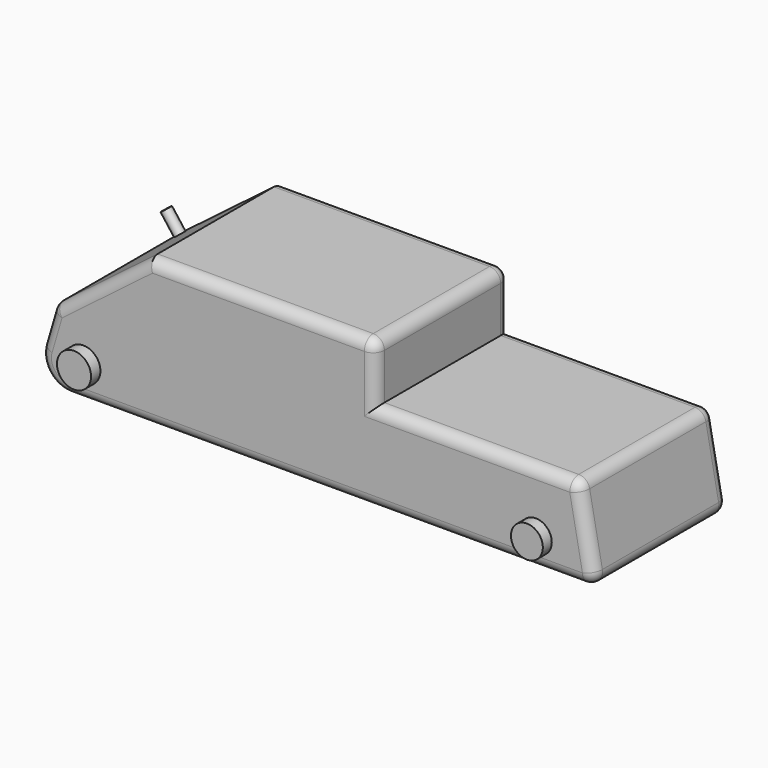
from build123d import *

# Parameters (mm, degrees)
F1_DEPTH    = 76.2
F2_R        = 5.08
F3_T1_DEPTH = 76.2
F3_T4_ANGLE = 106.3398594687
F3_T6_ANGLE = 106.3398594687
F4_R        = 7.7543468395
F5_DEPTH    = 0.254
F6_DEPTH    = 5.08
F7_R        = 7.6382634684
F8_DEPTH    = 5.08
F10_R       = 7.2706121331
F11_DEPTH   = 5.08
F9_R        = 7.2450103535
F12_DEPTH   = 5.08
F13_R       = 2.3168995741
F14_DEPTH   = 10.16


# Not quite as in the source:
# - a fillet or chamfer that OpenCascade refuses, or shapes differently, is made with other operations: its cross-section is extruded or revolved along the edge and cut away or added
# - the program builds the solid bodies; features that only make, move or delete a surface that nothing else refers to are left out


with BuildPart() as f1:
    # F0 (on Front) → F1 (new body)
    with BuildSketch(Plane.XZ):
        Polygon((-120.808057487, 0), (-130.5492073298, -33.2263112068), (126.3735592365, -33.2263112068), (118.6618208885, 7.3618022725), (26.1209160089, 7.3618022725), (26.1209160089, 33.3381965756), (-76.9728943706, 33.3381965756), align=None)
    extrude(amount=F1_DEPTH)

    # F2
    f2_edges = [f1.edges().sort_by_distance(p)[0] for p in [
        (-125.678632, -76.2, -16.613156),
        (-98.890476, -76.2, 16.669098),
        (-25.425989, -76.2, 33.338197),
        (26.120916, -76.2, 20.349999),
        (26.120916, 0, 20.349999),
        (26.120916, -38.1, 33.338197),
        (-98.890476, 0, 16.669098),
        (-25.425989, 0, 33.338197),
        (-125.678632, 0, -16.613156),
        (-2.087824, 0, -33.226311),
        (-120.808057, -38.1, 0),
        (-2.087824, -76.2, -33.226311),
        (72.391368, -76.2, 7.361802),
        (118.661821, -38.1, 7.361802),
        (122.51769, -76.2, -12.932254),
        (126.373559, -38.1, -33.226311),
        (122.51769, 0, -12.932254),
        (72.391368, 0, 7.361802),
    ]]
    fillet(f2_edges, radius=F2_R)

    # F3: fillet of radius 12.7 on 1 edges, made by hand

    # F3_s2 → F3_t1 (cut)
    with BuildSketch(Plane.XZ):
        with BuildLine():
            ThreePointArc((-125.7783735266, -16.9533648691), (-123.756623344, -28.1392469582), (-113.5913289929, -33.2263112068))
            Line((-113.5913289929, -33.2263112068), (-130.5492073298, -33.2263112068))
            Line((-130.5492073298, -33.2263112068), (-125.7783735266, -16.9533648691))
        make_face()
    extrude(amount=F3_T1_DEPTH, mode=Mode.SUBTRACT)

    # F3_s3 → F3_t4 (revolve, cut)
    with BuildSketch(Plane.YZ.offset(-113.5913289929)):
        with BuildLine():
            ThreePointArc((0, -28.1463112068), (-1.4878975516, -31.7384136552), (-5.08, -33.2263112068))
            Line((-5.08, -33.2263112068), (0, -33.2263112068))
            Line((0, -33.2263112068), (0, -28.1463112068))
        make_face()
    revolve(axis=Axis((-113.5913289929, 0, -20.5263112068), (0, 1, 0)), revolution_arc=F3_T4_ANGLE, mode=Mode.SUBTRACT)

    # F3_s5 → F3_t6 (revolve, cut)
    with BuildSketch(Plane(origin=(-14.5321554702, 0, -49.5680620824), x_dir=(0, 1, 0), z_dir=(0.2813343573, 0, 0.9596098058))):
        with BuildLine():
            ThreePointArc((-76.2, 110.848596585), (-74.7121024484, 114.4406990334), (-71.12, 115.928596585))
            Line((-71.12, 115.928596585), (-76.2, 115.928596585))
            Line((-76.2, 115.928596585), (-76.2, 110.848596585))
        make_face()
    revolve(axis=Axis((-113.5913289929, -76.2, -20.5263112068), (0, -1, 0)), revolution_arc=F3_T6_ANGLE, mode=Mode.SUBTRACT)

    # F4 (on face) → F5 (join)
    with BuildSketch(Plane.XZ.offset(76.2)):
        with Locations((-106.6796183586, -18.6145938933)):
            Circle(F4_R)
    extrude(amount=F5_DEPTH)

    # F6 (add): a face of the model
    f6_faces = [f1.faces().sort_by_distance(p)[0] for p in [
        (-106.6796183586, -76.454, -18.6145938933),
    ]]
    extrude(f6_faces, amount=F6_DEPTH)

    # F7 (on face) → F8 (join)
    with BuildSketch(Plane(origin=(0, 0, 0), x_dir=(-1, 0, 0), z_dir=(0, 1, 0))):
        with Locations((107.014529407, -18.2879995555)):
            Circle(F7_R)
    extrude(amount=F8_DEPTH)

    # F10 (on face) → F11 (join)
    with BuildSketch(Plane(origin=(0, 0, 0), x_dir=(-1, 0, 0), z_dir=(0, 1, 0))):
        with Locations((-98.7254753709, -20.7264013588)):
            Circle(F10_R)
    extrude(amount=F11_DEPTH)

    # F9 (on face) → F12 (join)
    with BuildSketch(Plane.XZ.offset(76.2)):
        with Locations((99.0302711725, -20.4215999693)):
            Circle(F9_R)
    extrude(amount=F12_DEPTH)

    # F13 (on face) → F14 (join)
    with BuildSketch(Plane(origin=(-44.2704434122, 0, 58.2095706289), x_dir=(0.7959568218, 0, 0.6053533991), z_dir=(-0.6053533991, 0, 0.7959568218))):
        with Locations((-89.274123311, -10.5928946286)):
            Circle(F13_R)
    extrude(amount=F14_DEPTH)


solid = f1.part
